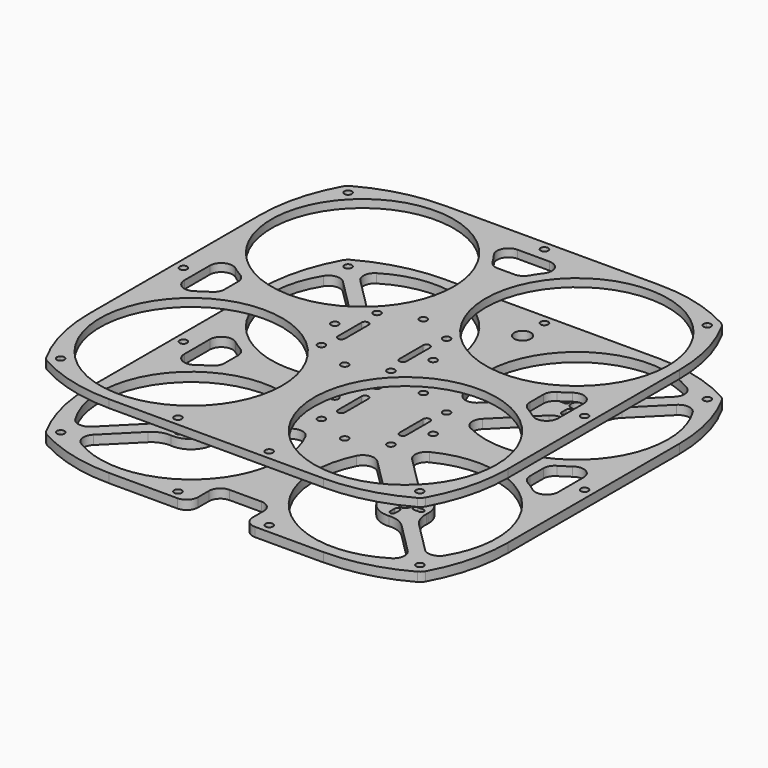
from build123d import *

# Parameters (mm, degrees)
F0_R     = 1.65
F0_W     = 3
F0_H     = 16
F1_DEPTH = 3.5
F2_R     = 5
F3_R     = 5
F4_R     = 1.49999
F6_R     = 1.65
F6_R_2   = 3.65
F6_R_3   = 2.5
F7_DEPTH = 4
F8_R     = 10
F9_R     = 5
F10_R    = 5
F11_R    = 5
F12_R    = 5
F13_R    = 5


# Not quite as in the source:
# - a fillet or chamfer is up to 0.001 mm smaller than in the source, because OpenCascade refuses the exact size


with BuildPart() as f1:
    # F0 (on Top) → F1 (new body)
    with BuildSketch(Plane.XY):
        with BuildLine():
            ThreePointArc((-118.3161303103, 11.4814622591), (-125.7425371815, 24.7657335065), (-128.3161303103, 39.7657335065))
            Line((-128.3161303103, 39.7657335065), (-128.3161303103, -54.2342664935))
            ThreePointArc((-128.3161303103, -54.2342664935), (-125.7425371815, -39.2342664935), (-118.3161303103, -25.949995246))
            Line((-118.3161303103, -25.949995246), (-118.3161303103, 11.4814622591))
        make_face()
        with Locations((-124.3161303103, -7.2342664935)):
            Circle(F0_R, mode=Mode.SUBTRACT)
        with BuildLine():
            ThreePointArc((-110.1359363333, 71.5855377903), (-110.5165386302, 69.6721207263), (-111.6004022776, 68.0500040342))
            ThreePointArc((-111.6004022776, 68.0500040342), (-114.9969936141, 66.587468671), (-118.4695912998, 67.8590455302))
            ThreePointArc((-118.4695912998, 67.8590455302), (-125.7832101753, 54.6501927757), (-128.3161303103, 39.7657335065))
            ThreePointArc((-128.3161303103, 39.7657335065), (-125.7425371815, 24.7657335065), (-118.3161303103, 11.4814622591))
            ThreePointArc((-118.3161303103, 11.4814622591), (-111.4659489145, 4.6575049476), (-103.3161303103, -0.545555235))
            ThreePointArc((-103.3161303103, -0.545555235), (-76.8540279471, -4.7678631711), (-52.6834054177, 6.8015686354))
            ThreePointArc((-52.6834054177, 6.8015686354), (-52.7328564993, 9.1824596955), (-50.3519654391, 9.1330086139))
            ThreePointArc((-50.3519654391, 9.1330086139), (-41.4330345603, 23.3095404353), (-38.3161303103, 39.7657335065))
            ThreePointArc((-38.3161303103, 39.7657335065), (-39.5039859131, 50.0368582413), (-43.0048415688, 59.7657335065))
            ThreePointArc((-43.0048415688, 59.7657335065), (-48.2079017513, 67.9155521107), (-55.0318590628, 74.7657335065))
            ThreePointArc((-55.0318590628, 74.7657335065), (-68.3161303103, 82.1921403777), (-83.3161303103, 84.7657335065))
            ThreePointArc((-83.3161303103, 84.7657335065), (-98.2005907401, 82.2328129648), (-111.4094442555, 74.9191929604))
            ThreePointArc((-111.4094442555, 74.9191929604), (-110.4651515819, 73.3698499281), (-110.1359363333, 71.5855377903))
        make_face()
        with BuildLine():
            ThreePointArc((-111.6004022776, 68.0500040342), (-68.0087934859, 76.7209150018), (-43.3161303103, 39.7657335065))
            ThreePointArc((-43.3161303103, 39.7657335065), (-98.6234671346, 2.8105520113), (-111.6004022776, 68.0500040342))
        make_face(mode=Mode.SUBTRACT)
        with BuildLine():
            ThreePointArc((-52.6834054177, 6.8015686354), (-76.8540279471, -4.7678631711), (-103.3161303103, -0.545555235))
            Line((-103.3161303103, -0.545555235), (-103.3161303103, -13.922977752))
            ThreePointArc((-103.3161303103, -13.922977752), (-76.8540279471, -9.7006698158), (-52.6834054177, -21.2701016223))
            ThreePointArc((-52.6834054177, -21.2701016223), (-50.9031838295, -20.9733058839), (-49.9161303103, -22.4842664935))
            ThreePointArc((-49.9161303103, -22.4842664935), (-50.028945865, -23.0839030345), (-50.3519654391, -23.6015416009))
            ThreePointArc((-50.3519654391, -23.6015416009), (-41.4330345603, -37.7780734222), (-38.3161303103, -54.2342664935))
            ThreePointArc((-38.3161303103, -54.2342664935), (-51.4963251569, -86.0540716469), (-83.3161303103, -99.2342664935))
            Line((-83.3161303103, -99.2342664935), (10.6838696897, -99.2342664935))
            ThreePointArc((10.6838696897, -99.2342664935), (-30.5682370454, -72.2138018022), (-22.2802951815, -23.6015416009))
            ThreePointArc((-22.2802951815, -23.6015416009), (-22.2328564993, -21.3175403045), (-19.9488552029, -21.2701016223))
            ThreePointArc((-19.9488552029, -21.2701016223), (4.2217673265, -9.7006698158), (30.6838696897, -13.922977752))
            Line((30.6838696897, -13.922977752), (30.6838696897, -0.545555235))
            ThreePointArc((30.6838696897, -0.545555235), (4.2217673265, -4.7678631711), (-19.9488552029, 6.8015686354))
            ThreePointArc((-19.9488552029, 6.8015686354), (-22.2328564993, 6.8490073176), (-22.2802951815, 9.1330086139))
            ThreePointArc((-22.2802951815, 9.1330086139), (-33.849726988, 33.3036311434), (-29.6274190518, 59.7657335065))
            Line((-29.6274190518, 59.7657335065), (-43.0048415688, 59.7657335065))
            ThreePointArc((-43.0048415688, 59.7657335065), (-39.5039859131, 50.0368582413), (-38.3161303103, 39.7657335065))
            ThreePointArc((-38.3161303103, 39.7657335065), (-41.4330345603, 23.3095404353), (-50.3519654391, 9.1330086139))
            ThreePointArc((-50.3519654391, 9.1330086139), (-50.028945865, 8.6153700475), (-49.9161303103, 8.0157335065))
            ThreePointArc((-49.9161303103, 8.0157335065), (-50.9031838295, 6.504772897), (-52.6834054177, 6.8015686354))
        make_face()
        with Locations((-56.3161303103, -95.2342664935)):
            Circle(F0_R, mode=Mode.SUBTRACT)
        with Locations((-16.3161303103, -95.2342664935)):
            Circle(F0_R, mode=Mode.SUBTRACT)
        with Locations((-36.3161303103, -28.8010226058)):
            Circle(F0_R, mode=Mode.SUBTRACT)
        with Locations((-57.8828868985, -7.2342664935)):
            Circle(F0_R, mode=Mode.SUBTRACT)
        with Locations((-49.8161303103, -7.2342664935)):
            Rectangle(F0_W, F0_H, mode=Mode.SUBTRACT)
        with Locations((-22.8161303103, -7.2342664935)):
            Rectangle(F0_W, F0_H, mode=Mode.SUBTRACT)
        with Locations((-14.7493727702, -7.2342664935)):
            Circle(F0_R, mode=Mode.SUBTRACT)
        with Locations((-36.3161303103, 14.3324905707)):
            Circle(F0_R, mode=Mode.SUBTRACT)
        with BuildLine():
            ThreePointArc((38.7771836349, 74.9191929604), (25.5683301195, 82.2328129648), (10.6838696897, 84.7657335065))
            ThreePointArc((10.6838696897, 84.7657335065), (-4.3161303103, 82.1921403777), (-17.6004015578, 74.7657335065))
            ThreePointArc((-17.6004015578, 74.7657335065), (-24.4243588693, 67.9155521107), (-29.6274190518, 59.7657335065))
            ThreePointArc((-29.6274190518, 59.7657335065), (-33.849726988, 33.3036311434), (-22.2802951815, 9.1330086139))
            ThreePointArc((-22.2802951815, 9.1330086139), (-20.4664937693, 9.5529179518), (-19.4161303103, 8.0157335065))
            ThreePointArc((-19.4161303103, 8.0157335065), (-19.5551697008, 7.3527870257), (-19.9488552029, 6.8015686354))
            ThreePointArc((-19.9488552029, 6.8015686354), (4.2217673265, -4.7678631711), (30.6838696897, -0.545555235))
            ThreePointArc((30.6838696897, -0.545555235), (38.8336882939, 4.6575049476), (45.6838696897, 11.4814622591))
            ThreePointArc((45.6838696897, 11.4814622591), (53.1102765609, 24.7657335065), (55.6838696897, 39.7657335065))
            ThreePointArc((55.6838696897, 39.7657335065), (53.1509495547, 54.6501927757), (45.8373306792, 67.8590455302))
            ThreePointArc((45.8373306792, 67.8590455302), (42.3647330544, 66.5874686693), (38.9681417432, 68.050003948))
            ThreePointArc((38.9681417432, 68.050003948), (37.5056065855, 71.4465953585), (38.7771836349, 74.9191929604))
        make_face()
        with BuildLine():
            ThreePointArc((50.6838696897, 39.7657335065), (-26.2713118289, 24.4583967385), (38.9681417432, 68.050003948))
            ThreePointArc((38.9681417432, 68.050003948), (47.6390512083, 55.0730702746), (50.6838696897, 39.7657335065))
        make_face(mode=Mode.SUBTRACT)
        with BuildLine():
            Line((55.6838696897, -54.2342664935), (55.6838696897, 39.7657335065))
            ThreePointArc((55.6838696897, 39.7657335065), (53.1102765609, 24.7657335065), (45.6838696897, 11.4814622591))
            Line((45.6838696897, 11.4814622591), (45.6838696897, -25.949995246))
            ThreePointArc((45.6838696897, -25.949995246), (53.1102765609, -39.2342664935), (55.6838696897, -54.2342664935))
        make_face()
        with Locations((51.6838696897, -7.2342664935)):
            Circle(F0_R, mode=Mode.SUBTRACT)
        with BuildLine():
            ThreePointArc((-118.3161303103, -25.949995246), (-125.7425371815, -39.2342664935), (-128.3161303103, -54.2342664935))
            ThreePointArc((-128.3161303103, -54.2342664935), (-125.7832101753, -69.1187257626), (-118.4695912998, -82.3275785171))
            ThreePointArc((-118.4695912998, -82.3275785171), (-114.9969936141, -81.056001658), (-111.6004022776, -82.5185370211))
            ThreePointArc((-111.6004022776, -82.5185370211), (-110.5165386302, -84.1406537133), (-110.1359363333, -86.0540707772))
            ThreePointArc((-110.1359363333, -86.0540707772), (-110.4651515819, -87.8383829151), (-111.4094442555, -89.3877259474))
            ThreePointArc((-111.4094442555, -89.3877259474), (-98.2005907401, -96.7013459517), (-83.3161303103, -99.2342664935))
            ThreePointArc((-83.3161303103, -99.2342664935), (-51.4963251569, -86.0540716469), (-38.3161303103, -54.2342664935))
            ThreePointArc((-38.3161303103, -54.2342664935), (-41.4330345603, -37.7780734222), (-50.3519654391, -23.6015416009))
            ThreePointArc((-50.3519654391, -23.6015416009), (-52.7328564993, -23.6509926824), (-52.6834054177, -21.2701016223))
            ThreePointArc((-52.6834054177, -21.2701016223), (-76.8540279471, -9.7006698158), (-103.3161303103, -13.922977752))
            ThreePointArc((-103.3161303103, -13.922977752), (-111.4659489145, -19.1260379345), (-118.3161303103, -25.949995246))
        make_face()
        with BuildLine():
            ThreePointArc((-43.3161303103, -54.2342664935), (-68.0087934859, -91.1894479887), (-111.6004022776, -82.5185370211))
            ThreePointArc((-111.6004022776, -82.5185370211), (-98.6234671346, -17.2790849982), (-43.3161303103, -54.2342664935))
        make_face(mode=Mode.SUBTRACT)
        with BuildLine():
            ThreePointArc((-22.2802951815, -23.6015416009), (-30.5682370454, -72.2138018022), (10.6838696897, -99.2342664935))
            ThreePointArc((10.6838696897, -99.2342664935), (25.5683301195, -96.7013459517), (38.7771836349, -89.3877259474))
            ThreePointArc((38.7771836349, -89.3877259474), (37.5056065853, -85.9151283522), (38.9681417336, -82.5185369445))
            ThreePointArc((38.9681417336, -82.5185369445), (42.3647330476, -81.0560016565), (45.8373306792, -82.3275785171))
            ThreePointArc((45.8373306792, -82.3275785171), (53.1509495547, -69.1187257626), (55.6838696897, -54.2342664935))
            ThreePointArc((55.6838696897, -54.2342664935), (53.1102765609, -39.2342664935), (45.6838696897, -25.949995246))
            ThreePointArc((45.6838696897, -25.949995246), (38.8336882939, -19.1260379345), (30.6838696897, -13.922977752))
            ThreePointArc((30.6838696897, -13.922977752), (4.2217673265, -9.7006698158), (-19.9488552029, -21.2701016223))
            ThreePointArc((-19.9488552029, -21.2701016223), (-19.5551697008, -21.8213200127), (-19.4161303103, -22.4842664935))
            ThreePointArc((-19.4161303103, -22.4842664935), (-20.4664937693, -24.0214509387), (-22.2802951815, -23.6015416009))
        make_face()
        with BuildLine():
            ThreePointArc((50.6838696897, -54.2342664935), (47.6390512057, -69.5416032678), (38.9681417336, -82.5185369445))
            ThreePointArc((38.9681417336, -82.5185369445), (-26.2713118263, -38.9269297191), (50.6838696897, -54.2342664935))
        make_face(mode=Mode.SUBTRACT)
        with BuildLine():
            Line((10.6838696897, 84.7657335065), (-83.3161303103, 84.7657335065))
            ThreePointArc((-83.3161303103, 84.7657335065), (-68.3161303103, 82.1921403777), (-55.0318590628, 74.7657335065))
            Line((-55.0318590628, 74.7657335065), (-17.6004015578, 74.7657335065))
            ThreePointArc((-17.6004015578, 74.7657335065), (-4.3161303103, 82.1921403777), (10.6838696897, 84.7657335065))
        make_face()
        with Locations((-36.3161303103, 80.7657335065)):
            Circle(F0_R, mode=Mode.SUBTRACT)
        with BuildLine():
            ThreePointArc((-118.4695912998, 67.8590455302), (-114.9969936141, 66.587468671), (-111.6004022776, 68.0500040342))
            ThreePointArc((-111.6004022776, 68.0500040342), (-110.5165386302, 69.6721207263), (-110.1359363333, 71.5855377903))
            ThreePointArc((-110.1359363333, 71.5855377903), (-110.4651515819, 73.3698499281), (-111.4094442555, 74.9191929604))
            ThreePointArc((-111.4094442555, 74.9191929604), (-112.6991130718, 73.8485785175), (-113.9480162869, 72.7306779403))
            ThreePointArc((-113.9480162869, 72.7306779403), (-113.6058108358, 72.202964678), (-113.4859363333, 71.5855377903))
            ThreePointArc((-113.4859363333, 71.5855377903), (-114.4905609156, 70.0669889533), (-116.2810764184, 70.3976176812))
            ThreePointArc((-116.2810764184, 70.3976176812), (-117.3989769273, 69.148714405), (-118.4695912998, 67.8590455302))
        make_face()
        with BuildLine():
            ThreePointArc((-117.5473543924, 75.9656134682), (-114.2956364532, 76.5144216509), (-111.4094442555, 74.9191929604))
            ThreePointArc((-111.4094442555, 74.9191929604), (-98.2005907401, 82.2328129648), (-83.3161303103, 84.7657335065))
            ThreePointArc((-83.3161303103, 84.7657335065), (-100.9882751635, 82.5305075258), (-117.5473543924, 75.9656134682))
        make_face()
        with BuildLine():
            ThreePointArc((-119.516012195, 73.9969555156), (-120.064820139, 70.7452375877), (-118.4695912998, 67.8590455302))
            ThreePointArc((-118.4695912998, 67.8590455302), (-117.3989769273, 69.148714405), (-116.2810764184, 70.3976176812))
            ThreePointArc((-116.2810764184, 70.3976176812), (-116.3026625542, 72.7522639473), (-113.9480162869, 72.7306779403))
            ThreePointArc((-113.9480162869, 72.7306779403), (-112.6991130718, 73.8485785175), (-111.4094442555, 74.9191929604))
            ThreePointArc((-111.4094442555, 74.9191929604), (-114.2956364532, 76.5144216509), (-117.5473543924, 75.9656134682))
            ThreePointArc((-117.5473543924, 75.9656134682), (-118.671470374, 75.1210715615), (-119.516012195, 73.9969555156))
        make_face()
        with BuildLine():
            ThreePointArc((-128.3161303103, 39.7657335065), (-125.7832101753, 54.6501927757), (-118.4695912998, 67.8590455302))
            ThreePointArc((-118.4695912998, 67.8590455302), (-120.064820139, 70.7452375877), (-119.516012195, 73.9969555156))
            ThreePointArc((-119.516012195, 73.9969555156), (-126.0809048288, 57.4378771164), (-128.3161303103, 39.7657335065))
        make_face()
        with BuildLine():
            ThreePointArc((55.6838696897, 39.7657335065), (53.4486442082, 57.4378771164), (46.8837515744, 73.9969555156))
            ThreePointArc((46.8837515744, 73.9969555156), (47.3462153, 72.8304515808), (47.5036757128, 71.5855377903))
            ThreePointArc((47.5036757128, 71.5855377903), (47.0681184406, 69.5444933067), (45.8373306792, 67.8590455302))
            ThreePointArc((45.8373306792, 67.8590455302), (53.1509495547, 54.6501927757), (55.6838696897, 39.7657335065))
        make_face()
        with BuildLine():
            ThreePointArc((44.9150937718, 75.9656134682), (41.6633758326, 76.5144216509), (38.7771836349, 74.9191929604))
            ThreePointArc((38.7771836349, 74.9191929604), (40.0668524512, 73.8485785175), (41.3157556663, 72.7306779403))
            ThreePointArc((41.3157556663, 72.7306779403), (43.1211026004, 73.1156632879), (44.1536757128, 71.5855377903))
            ThreePointArc((44.1536757128, 71.5855377903), (44.0222245497, 70.9401623725), (43.6488157978, 70.3976176812))
            ThreePointArc((43.6488157978, 70.3976176812), (44.7667163068, 69.148714405), (45.8373306792, 67.8590455302))
            ThreePointArc((45.8373306792, 67.8590455302), (47.0681184406, 69.5444933067), (47.5036757128, 71.5855377903))
            ThreePointArc((47.5036757128, 71.5855377903), (47.3462153, 72.8304515808), (46.8837515744, 73.9969555156))
            ThreePointArc((46.8837515744, 73.9969555156), (46.0392097534, 75.1210715615), (44.9150937718, 75.9656134682))
        make_face()
        with BuildLine():
            ThreePointArc((44.9150937718, 75.9656134682), (28.3560145429, 82.5305075258), (10.6838696897, 84.7657335065))
            ThreePointArc((10.6838696897, 84.7657335065), (25.5683301195, 82.2328129648), (38.7771836349, 74.9191929604))
            ThreePointArc((38.7771836349, 74.9191929604), (41.6633758326, 76.5144216509), (44.9150937718, 75.9656134682))
        make_face()
        with BuildLine():
            ThreePointArc((41.3157556663, 72.7306779403), (40.0668524512, 73.8485785175), (38.7771836349, 74.9191929604))
            ThreePointArc((38.7771836349, 74.9191929604), (37.5056065855, 71.4465953585), (38.9681417432, 68.050003948))
            ThreePointArc((38.9681417432, 68.050003948), (42.3647330544, 66.5874686693), (45.8373306792, 67.8590455302))
            ThreePointArc((45.8373306792, 67.8590455302), (44.7667163068, 69.148714405), (43.6488157978, 70.3976176812))
            ThreePointArc((43.6488157978, 70.3976176812), (41.3369494919, 70.4188116332), (41.3157556663, 72.7306779403))
        make_face()
        with BuildLine():
            ThreePointArc((41.3157556663, -87.1992109272), (40.0668524512, -88.3171115044), (38.7771836349, -89.3877259474))
            ThreePointArc((38.7771836349, -89.3877259474), (41.6633758326, -90.9829546378), (44.9150937718, -90.4341464552))
            ThreePointArc((44.9150937718, -90.4341464552), (46.0392097534, -89.5896045485), (46.8837515744, -88.4654885026))
            ThreePointArc((46.8837515744, -88.4654885026), (47.3462153, -87.2989845677), (47.5036757128, -86.0540707772))
            ThreePointArc((47.5036757128, -86.0540707772), (47.0681184406, -84.0130262937), (45.8373306792, -82.3275785171))
            ThreePointArc((45.8373306792, -82.3275785171), (44.7667163068, -83.6172473919), (43.6488157978, -84.8661506681))
            ThreePointArc((43.6488157978, -84.8661506681), (44.0222245497, -85.4086953595), (44.1536757128, -86.0540707772))
            ThreePointArc((44.1536757128, -86.0540707772), (43.1211026004, -87.5841962748), (41.3157556663, -87.1992109272))
        make_face()
        with BuildLine():
            ThreePointArc((46.8837515744, -88.4654885026), (53.4486442082, -71.9064101034), (55.6838696897, -54.2342664935))
            ThreePointArc((55.6838696897, -54.2342664935), (53.1509495547, -69.1187257626), (45.8373306792, -82.3275785171))
            ThreePointArc((45.8373306792, -82.3275785171), (47.0681184406, -84.0130262937), (47.5036757128, -86.0540707772))
            ThreePointArc((47.5036757128, -86.0540707772), (47.3462153, -87.2989845677), (46.8837515744, -88.4654885026))
        make_face()
        with BuildLine():
            ThreePointArc((38.9681417336, -82.5185369445), (37.5056065853, -85.9151283522), (38.7771836349, -89.3877259474))
            ThreePointArc((38.7771836349, -89.3877259474), (40.0668524512, -88.3171115044), (41.3157556663, -87.1992109272))
            ThreePointArc((41.3157556663, -87.1992109272), (41.3369494919, -84.8873446201), (43.6488157978, -84.8661506681))
            ThreePointArc((43.6488157978, -84.8661506681), (44.7667163068, -83.6172473919), (45.8373306792, -82.3275785171))
            ThreePointArc((45.8373306792, -82.3275785171), (42.3647330476, -81.0560016565), (38.9681417336, -82.5185369445))
        make_face()
        with BuildLine():
            ThreePointArc((38.7771836349, -89.3877259474), (25.5683301195, -96.7013459517), (10.6838696897, -99.2342664935))
            ThreePointArc((10.6838696897, -99.2342664935), (28.3560145429, -96.9990405127), (44.9150937718, -90.4341464552))
            ThreePointArc((44.9150937718, -90.4341464552), (41.6633758326, -90.9829546378), (38.7771836349, -89.3877259474))
        make_face()
        with BuildLine():
            ThreePointArc((-111.4094442555, -89.3877259474), (-114.2956364532, -90.9829546378), (-117.5473543924, -90.4341464552))
            ThreePointArc((-117.5473543924, -90.4341464552), (-100.9882751635, -96.9990405127), (-83.3161303103, -99.2342664935))
            ThreePointArc((-83.3161303103, -99.2342664935), (-98.2005907401, -96.7013459517), (-111.4094442555, -89.3877259474))
        make_face()
        with BuildLine():
            ThreePointArc((-116.2810764184, -84.8661506681), (-117.3989769273, -83.6172473919), (-118.4695912998, -82.3275785171))
            ThreePointArc((-118.4695912998, -82.3275785171), (-120.064820139, -85.2137705746), (-119.516012195, -88.4654885026))
            ThreePointArc((-119.516012195, -88.4654885026), (-118.671470374, -89.5896045485), (-117.5473543924, -90.4341464552))
            ThreePointArc((-117.5473543924, -90.4341464552), (-114.2956364532, -90.9829546378), (-111.4094442555, -89.3877259474))
            ThreePointArc((-111.4094442555, -89.3877259474), (-112.6991130718, -88.3171115044), (-113.9480162869, -87.1992109272))
            ThreePointArc((-113.9480162869, -87.1992109272), (-116.3026625542, -87.2207969343), (-116.2810764184, -84.8661506681))
        make_face()
        with BuildLine():
            ThreePointArc((-111.6004022776, -82.5185370211), (-114.9969936141, -81.056001658), (-118.4695912998, -82.3275785171))
            ThreePointArc((-118.4695912998, -82.3275785171), (-117.3989769273, -83.6172473919), (-116.2810764184, -84.8661506681))
            ThreePointArc((-116.2810764184, -84.8661506681), (-114.4905609156, -84.5355219403), (-113.4859363333, -86.0540707772))
            ThreePointArc((-113.4859363333, -86.0540707772), (-113.6058108358, -86.6714976649), (-113.9480162869, -87.1992109272))
            ThreePointArc((-113.9480162869, -87.1992109272), (-112.6991130718, -88.3171115044), (-111.4094442555, -89.3877259474))
            ThreePointArc((-111.4094442555, -89.3877259474), (-110.4651515819, -87.8383829151), (-110.1359363333, -86.0540707772))
            ThreePointArc((-110.1359363333, -86.0540707772), (-110.5165386302, -84.1406537133), (-111.6004022776, -82.5185370211))
        make_face()
        with BuildLine():
            ThreePointArc((-118.4695912998, -82.3275785171), (-125.7832101753, -69.1187257626), (-128.3161303103, -54.2342664935))
            ThreePointArc((-128.3161303103, -54.2342664935), (-126.0809048288, -71.9064101034), (-119.516012195, -88.4654885026))
            ThreePointArc((-119.516012195, -88.4654885026), (-120.064820139, -85.2137705746), (-118.4695912998, -82.3275785171))
        make_face()
    extrude(amount=F1_DEPTH)

    # F2
    f2_edges = [f1.edges().sort_by_distance(p)[0] for p in [
        (-118.31613, 11.481462, 1.75),
        (45.68387, 11.481462, 1.75),
        (45.68387, -25.949995, 1.75),
        (-118.31613, -25.949995, 1.75),
        (-17.600402, 74.765734, 1.75),
        (-55.031859, 74.765734, 1.75),
    ]]
    fillet(f2_edges, radius=F2_R)

    # F3
    f3_edges = [f1.edges().sort_by_distance(p)[0] for p in [
        (30.68387, -0.545555, 1.75),
        (30.68387, -13.922978, 1.75),
        (-103.31613, -0.545555, 1.75),
        (-103.31613, -13.922978, 1.75),
        (-29.627419, 59.765734, 1.75),
        (-43.004842, 59.765734, 1.75),
    ]]
    fillet(f3_edges, radius=F3_R)

    # F4 (radius 1.5 in the source; OpenCascade refuses exactly that, so slightly less here)
    f4_edges = [f1.edges().sort_by_distance(p)[0] for p in [
        (-51.31613, -15.234266, 1.75),
        (-24.31613, -15.234266, 1.75),
        (-48.31613, -15.234266, 1.75),
        (-21.31613, -15.234266, 1.75),
        (-24.31613, 0.765734, 1.75),
        (-51.31613, 0.765734, 1.75),
        (-21.31613, 0.765734, 1.75),
        (-48.31613, 0.765734, 1.75),
    ]]
    fillet(f4_edges, radius=F4_R)


with BuildPart() as f7:
    # F6 (on offset) → F7 (new body)
    with BuildSketch(Plane(origin=(0, 0, -25), x_dir=(1, 0, 0), z_dir=(0, 0, -1))):
        with BuildLine():
            ThreePointArc((-110.3161303103, 18.2342664935), (-123.5653539053, 34.109654696), (-128.3161303103, 54.2342664935))
            Line((-128.3161303103, 54.2342664935), (-128.3161303103, -39.7657335065))
            ThreePointArc((-128.3161303103, -39.7657335065), (-126.0809048288, -57.4378771164), (-119.516012195, -73.9969555156))
            ThreePointArc((-119.516012195, -73.9969555156), (-118.1392463202, -67.5880224216), (-111.6004023308, -68.0500039809))
            ThreePointArc((-111.6004023308, -68.0500039809), (-110.5165386447, -69.6721206915), (-110.1359363333, -71.5855377903))
            ThreePointArc((-110.1359363333, -71.5855377903), (-112.5920309003, -75.8900174508), (-117.5473543924, -75.9656134682))
            ThreePointArc((-117.5473543924, -75.9656134682), (-100.9882751635, -82.5305075258), (-83.3161303103, -84.7657335065))
            Line((-83.3161303103, -84.7657335065), (10.6838696897, -84.7657335065))
            ThreePointArc((10.6838696897, -84.7657335065), (28.3560145429, -82.5305075258), (44.9150937718, -75.9656134682))
            ThreePointArc((44.9150937718, -75.9656134682), (38.5061605306, -74.5888480254), (38.9681417336, -68.0500039576))
            ThreePointArc((38.9681417336, -68.0500039576), (44.4170928267, -66.9661401079), (47.5036757128, -71.5855377903))
            ThreePointArc((47.5036757128, -71.5855377903), (47.3462153, -72.8304515808), (46.8837515744, -73.9969555156))
            ThreePointArc((46.8837515744, -73.9969555156), (53.4486442082, -57.4378771164), (55.6838696897, -39.7657335065))
            Line((55.6838696897, -39.7657335065), (55.6838696897, 54.2342664935))
            ThreePointArc((55.6838696897, 54.2342664935), (53.1509495547, 69.1187257626), (45.8373306792, 82.3275785171))
            ThreePointArc((45.8373306792, 82.3275785171), (42.364732999, 81.0560016578), (38.9681416648, 82.5185370133))
            ThreePointArc((38.9681416648, 82.5185370133), (37.505606584, 85.9151284009), (38.7771836349, 89.3877259474))
            ThreePointArc((38.7771836349, 89.3877259474), (25.5683301195, 96.7013459517), (10.6838696897, 99.2342664935))
            Line((10.6838696897, 99.2342664935), (-24.3161303103, 99.2342664935))
            Line((-24.3161303103, 99.2342664935), (-24.3161303103, 83.2342664935))
            Line((-24.3161303103, 83.2342664935), (-36.3161303103, 83.2342664935))
            Line((-36.3161303103, 83.2342664935), (-48.3161303103, 83.2342664935))
            Line((-48.3161303103, 83.2342664935), (-48.3161303103, 99.2342664935))
            Line((-48.3161303103, 99.2342664935), (-83.3161303103, 99.2342664935))
            ThreePointArc((-83.3161303103, 99.2342664935), (-51.4963251569, 86.0540716469), (-38.3161303103, 54.2342664935))
            ThreePointArc((-38.3161303103, 54.2342664935), (-41.4330345603, 37.7780734222), (-50.3519654391, 23.6015416009))
            ThreePointArc((-50.3519654391, 23.6015416009), (-50.028945865, 23.0839030345), (-49.9161303103, 22.4842664935))
            ThreePointArc((-49.9161303103, 22.4842664935), (-50.9031838295, 20.9733058839), (-52.6834054177, 21.2701016223))
            ThreePointArc((-52.6834054177, 21.2701016223), (-78.2608112683, 9.5191264469), (-105.8161303103, 15.2631233232))
            ThreePointArc((-105.8161303103, 15.2631233232), (-103.9860032914, 13.4329963042), (-103.3161303103, 10.9329963042))
            Line((-103.3161303103, 10.9329963042), (-103.3161303103, 3.5355366827))
            ThreePointArc((-103.3161303103, 3.5355366827), (-103.9860032914, 1.0355366827), (-105.8161303103, -0.7945903362))
            ThreePointArc((-105.8161303103, -0.7945903362), (-108.1106745274, -2.2126966511), (-110.3161303103, -3.7657335065))
            ThreePointArc((-110.3161303103, -3.7657335065), (-115.5521982878, -4.2378694615), (-118.3161303103, 0.2342664935))
            Line((-118.3161303103, 0.2342664935), (-118.3161303103, 14.2342664935))
            ThreePointArc((-118.3161303103, 14.2342664935), (-115.5521982878, 18.7064024485), (-110.3161303103, 18.2342664935))
        make_face()
        with BuildLine():
            ThreePointArc((-109.3994195191, -70.0916634024), (-110.5190717285, -69.091489732), (-111.6004023308, -68.0500039809))
            ThreePointArc((-111.6004023308, -68.0500039809), (-112.6418872793, -66.9686741232), (-113.6420602062, -65.8490227153))
            ThreePointArc((-113.6420602062, -65.8490227153), (-112.647698019, -12.5690584202), (-59.5945080892, -7.5588299112))
            ThreePointArc((-59.5945080892, -7.5588299112), (-55.0318590628, -11.4814622591), (-51.109226715, -16.0441112854))
            ThreePointArc((-51.109226715, -16.0441112854), (-45.3143136181, -27.2812660332), (-43.3161303103, -39.7657335065))
            ThreePointArc((-43.3161303103, -39.7657335065), (-66.6327788537, -76.120455128), (-109.3994195191, -70.0916634024))
        make_face(mode=Mode.SUBTRACT)
        with Locations((-51.5661303103, -8.0157335065)):
            Circle(F6_R, mode=Mode.SUBTRACT)
        with Locations((-57.8828868985, 7.2342664935)):
            Circle(F6_R, mode=Mode.SUBTRACT)
        with Locations((-36.3161303103, -80.7657335065)):
            Circle(F6_R, mode=Mode.SUBTRACT)
        with Locations((-36.3161303103, -68.7657335065)):
            Circle(F6_R_2, mode=Mode.SUBTRACT)
        with BuildLine():
            ThreePointArc((41.0097995856, -65.8490227153), (40.0096266699, -66.9686741111), (38.9681417336, -68.0500039576))
            ThreePointArc((38.9681417336, -68.0500039576), (37.88681112, -69.0914897208), (36.7671588985, -70.0916634024))
            ThreePointArc((36.7671588985, -70.0916634024), (-16.5128053966, -69.0973012153), (-21.5230339056, -16.0441112854))
            ThreePointArc((-21.5230339056, -16.0441112854), (-17.6004015578, -11.4814622591), (-13.0377525314, -7.5588299112))
            ThreePointArc((-13.0377525314, -7.5588299112), (28.7273603602, -4.0665396162), (50.6838696897, -39.7657335065))
            ThreePointArc((50.6838696897, -39.7657335065), (48.1874508243, -53.6754927454), (41.0097995856, -65.8490227153))
        make_face(mode=Mode.SUBTRACT)
        with Locations((-36.3161303103, -14.3324905707)):
            Circle(F6_R, mode=Mode.SUBTRACT)
        with Locations((-21.0661303103, -8.0157335065)):
            Circle(F6_R, mode=Mode.SUBTRACT)
        with Locations((-14.7493727702, 7.2342664935)):
            Circle(F6_R, mode=Mode.SUBTRACT)
        with Locations((51.6838696897, 7.2342664935)):
            Circle(F6_R, mode=Mode.SUBTRACT)
        with Locations((-124.3161303103, 7.2342664935)):
            Circle(F6_R, mode=Mode.SUBTRACT)
        with BuildLine():
            ThreePointArc((-51.3161303103, 13.7342664935), (-49.8161303103, 15.2342664935), (-48.3161303103, 13.7342664935))
            Line((-48.3161303103, 13.7342664935), (-48.3161303103, 0.7342664935))
            ThreePointArc((-48.3161303103, 0.7342664935), (-49.8161303103, -0.7657335065), (-51.3161303103, 0.7342664935))
            Line((-51.3161303103, 0.7342664935), (-51.3161303103, 13.7342664935))
        make_face(mode=Mode.SUBTRACT)
        with Locations((-56.3161303103, 95.2342664935)):
            Circle(F6_R, mode=Mode.SUBTRACT)
        with BuildLine():
            ThreePointArc((-24.3161303103, 13.7342664935), (-22.8161303103, 15.2342664935), (-21.3161303103, 13.7342664935))
            Line((-21.3161303103, 13.7342664935), (-21.3161303103, 0.7342664935))
            ThreePointArc((-21.3161303103, 0.7342664935), (-22.8161303103, -0.7657335065), (-24.3161303103, 0.7342664935))
            Line((-24.3161303103, 0.7342664935), (-24.3161303103, 13.7342664935))
        make_face(mode=Mode.SUBTRACT)
        with Locations((-36.3161303103, 28.8010226058)):
            Circle(F6_R, mode=Mode.SUBTRACT)
        with Locations((-21.0661303103, 22.4842664935)):
            Circle(F6_R, mode=Mode.SUBTRACT)
        with BuildLine():
            ThreePointArc((37.6838696897, 18.2342664935), (42.9199376672, 18.7064024485), (45.6838696897, 14.2342664935))
            Line((45.6838696897, 14.2342664935), (45.6838696897, 0.2342664935))
            ThreePointArc((45.6838696897, 0.2342664935), (42.9199376672, -4.2378694615), (37.6838696897, -3.7657335065))
            ThreePointArc((37.6838696897, -3.7657335065), (35.4784139068, -2.2126966511), (33.1838696897, -0.7945903362))
            ThreePointArc((33.1838696897, -0.7945903362), (31.3537426708, 1.0355366827), (30.6838696897, 3.5355366827))
            Line((30.6838696897, 3.5355366827), (30.6838696897, 10.9329963042))
            ThreePointArc((30.6838696897, 10.9329963042), (31.3537426708, 13.4329963042), (33.1838696897, 15.2631233232))
            ThreePointArc((33.1838696897, 15.2631233232), (35.4784139068, 16.681229638), (37.6838696897, 18.2342664935))
        make_face(mode=Mode.SUBTRACT)
        with Locations((-16.3161303103, 95.2342664935)):
            Circle(F6_R, mode=Mode.SUBTRACT)
        with BuildLine():
            ThreePointArc((36.7671588985, 84.5601963894), (37.8868110844, 83.5600227408), (38.9681416648, 82.5185370133))
            ThreePointArc((38.9681416648, 82.5185370133), (40.0096266368, 81.4372071337), (41.0097995856, 80.3175557023))
            ThreePointArc((41.0097995856, 80.3175557023), (48.1874508243, 68.1440257323), (50.6838696897, 54.2342664935))
            ThreePointArc((50.6838696897, 54.2342664935), (28.7273603602, 18.5350726031), (-13.0377525314, 22.0273628981))
            ThreePointArc((-13.0377525314, 22.0273628981), (-17.6004015578, 25.949995246), (-21.5230339056, 30.5126442724))
            ThreePointArc((-21.5230339056, 30.5126442724), (-16.5128053966, 83.5658342022), (36.7671588985, 84.5601963894))
        make_face(mode=Mode.SUBTRACT)
        with BuildLine():
            ThreePointArc((-118.4695912998, 82.3275785171), (-125.7832101753, 69.1187257626), (-128.3161303103, 54.2342664935))
            ThreePointArc((-128.3161303103, 54.2342664935), (-123.5653539053, 34.109654696), (-110.3161303103, 18.2342664935))
            ThreePointArc((-110.3161303103, 18.2342664935), (-108.1106745274, 16.681229638), (-105.8161303103, 15.2631233232))
            ThreePointArc((-105.8161303103, 15.2631233232), (-78.2608112683, 9.5191264469), (-52.6834054177, 21.2701016223))
            ThreePointArc((-52.6834054177, 21.2701016223), (-52.7328564993, 23.6509926824), (-50.3519654391, 23.6015416009))
            ThreePointArc((-50.3519654391, 23.6015416009), (-41.4330345603, 37.7780734222), (-38.3161303103, 54.2342664935))
            ThreePointArc((-38.3161303103, 54.2342664935), (-51.4963251569, 86.0540716469), (-83.3161303103, 99.2342664935))
            ThreePointArc((-83.3161303103, 99.2342664935), (-98.2005907401, 96.7013459517), (-111.4094442555, 89.3877259474))
            ThreePointArc((-111.4094442555, 89.3877259474), (-110.4651515819, 87.8383829151), (-110.1359363333, 86.0540707772))
            ThreePointArc((-110.1359363333, 86.0540707772), (-110.5165386423, 84.1406536843), (-111.6004023219, 82.5185369767))
            ThreePointArc((-111.6004023219, 82.5185369767), (-114.9969936454, 81.0560016571), (-118.4695912998, 82.3275785171))
        make_face()
        with BuildLine():
            ThreePointArc((-113.6420602062, 80.3175557023), (-112.641887275, 81.4372071148), (-111.6004023219, 82.5185369767))
            ThreePointArc((-111.6004023219, 82.5185369767), (-110.5190717239, 83.5600227232), (-109.3994195191, 84.5601963894))
            ThreePointArc((-109.3994195191, 84.5601963894), (-66.6327788537, 90.588988115), (-43.3161303103, 54.2342664935))
            ThreePointArc((-43.3161303103, 54.2342664935), (-45.3143136181, 41.7497990201), (-51.109226715, 30.5126442724))
            ThreePointArc((-51.109226715, 30.5126442724), (-55.0318590628, 25.949995246), (-59.5945080892, 22.0273628981))
            ThreePointArc((-59.5945080892, 22.0273628981), (-112.647698019, 27.0375914072), (-113.6420602062, 80.3175557023))
        make_face(mode=Mode.SUBTRACT)
        with BuildLine():
            Line((0.7843747531, 52.8200529311), (-21.5230339056, 30.5126442724))
            ThreePointArc((-21.5230339056, 30.5126442724), (-17.6004015578, 25.949995246), (-13.0377525314, 22.0273628981))
            Line((-13.0377525314, 22.0273628981), (9.2696561273, 44.3347715569))
            ThreePointArc((9.2696561273, 44.3347715569), (3.6128018778, 47.1631986816), (0.7843747531, 52.8200529311))
        make_face()
        with BuildLine():
            Line((-81.9019167479, 44.3347715569), (-59.5945080892, 22.0273628981))
            ThreePointArc((-59.5945080892, 22.0273628981), (-55.0318590628, 25.949995246), (-51.109226715, 30.5126442724))
            Line((-51.109226715, 30.5126442724), (-73.4166353737, 52.8200529311))
            ThreePointArc((-73.4166353737, 52.8200529311), (-76.2450624984, 47.1631986816), (-81.9019167479, 44.3347715569))
        make_face()
        with BuildLine():
            ThreePointArc((-51.109226715, -16.0441112854), (-55.0318590628, -11.4814622591), (-59.5945080892, -7.5588299112))
            Line((-59.5945080892, -7.5588299112), (-81.9019167479, -29.8662385699))
            ThreePointArc((-81.9019167479, -29.8662385699), (-76.2450624984, -32.6946656947), (-73.4166353737, -38.3515199442))
            Line((-73.4166353737, -38.3515199442), (-51.109226715, -16.0441112854))
        make_face()
        with BuildLine():
            ThreePointArc((-13.0377525314, -7.5588299112), (-17.6004015578, -11.4814622591), (-21.5230339056, -16.0441112854))
            Line((-21.5230339056, -16.0441112854), (0.7843747531, -38.3515199442))
            ThreePointArc((0.7843747531, -38.3515199442), (3.6128018778, -32.6946656947), (9.2696561273, -29.8662385699))
            Line((9.2696561273, -29.8662385699), (-13.0377525314, -7.5588299112))
        make_face()
        with BuildLine():
            ThreePointArc((20.6838696897, 54.2342664935), (20.3964103267, 56.61471905), (19.5505588149, 58.8583149315))
            ThreePointArc((19.5505588149, 58.8583149315), (17.7549375016, 61.3053343053), (15.3079181278, 63.1009556186))
            ThreePointArc((15.3079181278, 63.1009556186), (4.9061691127, 62.3962623304), (0.7843747531, 52.8200529311))
            ThreePointArc((0.7843747531, 52.8200529311), (3.6128018778, 47.1631986816), (9.2696561273, 44.3347715569))
            ThreePointArc((9.2696561273, 44.3347715569), (17.2358871033, 46.6797269435), (20.6838696897, 54.2342664935))
        make_face()
        with BuildLine():
            Line((11.7838696897, 49.7342664935), (11.7838696897, 47.2342664935))
            ThreePointArc((11.7838696897, 47.2342664935), (10.6838696897, 46.1342664935), (9.5838696897, 47.2342664935))
            Line((9.5838696897, 47.2342664935), (9.5838696897, 49.7342664935))
            ThreePointArc((9.5838696897, 49.7342664935), (10.6838696897, 50.8342664935), (11.7838696897, 49.7342664935))
        make_face(mode=Mode.SUBTRACT)
        with BuildLine():
            ThreePointArc((6.1838696897, 55.3342664935), (6.961687149, 55.0120839528), (7.2838696897, 54.2342664935))
            ThreePointArc((7.2838696897, 54.2342664935), (6.961687149, 53.4564490342), (6.1838696897, 53.1342664935))
            Line((6.1838696897, 53.1342664935), (3.6838696897, 53.1342664935))
            ThreePointArc((3.6838696897, 53.1342664935), (2.5838696897, 54.2342664935), (3.6838696897, 55.3342664935))
            Line((3.6838696897, 55.3342664935), (6.1838696897, 55.3342664935))
        make_face(mode=Mode.SUBTRACT)
        with Locations((10.6838696897, 54.2342664935)):
            Circle(F6_R_3, mode=Mode.SUBTRACT)
        with BuildLine():
            Line((15.1838696897, 55.3342664935), (17.6838696897, 55.3342664935))
            ThreePointArc((17.6838696897, 55.3342664935), (18.461687149, 55.0120839528), (18.7838696897, 54.2342664935))
            ThreePointArc((18.7838696897, 54.2342664935), (18.461687149, 53.4564490342), (17.6838696897, 53.1342664935))
            Line((17.6838696897, 53.1342664935), (15.1838696897, 53.1342664935))
            ThreePointArc((15.1838696897, 53.1342664935), (14.0838696897, 54.2342664935), (15.1838696897, 55.3342664935))
        make_face(mode=Mode.SUBTRACT)
        with BuildLine():
            Line((11.7838696897, 61.2342664935), (11.7838696897, 58.7342664935))
            ThreePointArc((11.7838696897, 58.7342664935), (10.6838696897, 57.6342664935), (9.5838696897, 58.7342664935))
            Line((9.5838696897, 58.7342664935), (9.5838696897, 61.2342664935))
            ThreePointArc((9.5838696897, 61.2342664935), (10.6838696897, 62.3342664935), (11.7838696897, 61.2342664935))
        make_face(mode=Mode.SUBTRACT)
        with BuildLine():
            ThreePointArc((-73.3161303103, 54.2342664935), (-78.1315611084, 62.7853039855), (-87.9401787484, 63.1009556186))
            ThreePointArc((-87.9401787484, 63.1009556186), (-90.3871981222, 61.3053343053), (-92.1828194355, 58.8583149315))
            ThreePointArc((-92.1828194355, 58.8583149315), (-91.4781261473, 48.4565659165), (-81.9019167479, 44.3347715569))
            ThreePointArc((-81.9019167479, 44.3347715569), (-76.2450624984, 47.1631986816), (-73.4166353737, 52.8200529311))
            ThreePointArc((-73.4166353737, 52.8200529311), (-73.3412882222, 53.5253762926), (-73.3161303103, 54.2342664935))
        make_face()
        with BuildLine():
            ThreePointArc((-82.2161303103, 47.2342664935), (-83.3161303103, 46.1342664935), (-84.4161303103, 47.2342664935))
            Line((-84.4161303103, 47.2342664935), (-84.4161303103, 49.7342664935))
            ThreePointArc((-84.4161303103, 49.7342664935), (-83.3161303103, 50.8342664935), (-82.2161303103, 49.7342664935))
            Line((-82.2161303103, 49.7342664935), (-82.2161303103, 47.2342664935))
        make_face(mode=Mode.SUBTRACT)
        with BuildLine():
            ThreePointArc((-87.8161303103, 55.3342664935), (-87.038312851, 55.0120839528), (-86.7161303103, 54.2342664935))
            ThreePointArc((-86.7161303103, 54.2342664935), (-87.038312851, 53.4564490342), (-87.8161303103, 53.1342664935))
            Line((-87.8161303103, 53.1342664935), (-90.3161303103, 53.1342664935))
            ThreePointArc((-90.3161303103, 53.1342664935), (-91.4161303103, 54.2342664935), (-90.3161303103, 55.3342664935))
            Line((-90.3161303103, 55.3342664935), (-87.8161303103, 55.3342664935))
        make_face(mode=Mode.SUBTRACT)
        with Locations((-83.3161303103, 54.2342664935)):
            Circle(F6_R_3, mode=Mode.SUBTRACT)
        with BuildLine():
            ThreePointArc((-84.4161303103, 61.2342664935), (-83.3161303103, 62.3342664935), (-82.2161303103, 61.2342664935))
            Line((-82.2161303103, 61.2342664935), (-82.2161303103, 58.7342664935))
            ThreePointArc((-82.2161303103, 58.7342664935), (-83.3161303103, 57.6342664935), (-84.4161303103, 58.7342664935))
            Line((-84.4161303103, 58.7342664935), (-84.4161303103, 61.2342664935))
        make_face(mode=Mode.SUBTRACT)
        with BuildLine():
            ThreePointArc((-75.2161303103, 54.2342664935), (-75.538312851, 53.4564490342), (-76.3161303103, 53.1342664935))
            Line((-76.3161303103, 53.1342664935), (-78.8161303103, 53.1342664935))
            ThreePointArc((-78.8161303103, 53.1342664935), (-79.9161303103, 54.2342664935), (-78.8161303103, 55.3342664935))
            Line((-78.8161303103, 55.3342664935), (-76.3161303103, 55.3342664935))
            ThreePointArc((-76.3161303103, 55.3342664935), (-75.538312851, 55.0120839528), (-75.2161303103, 54.2342664935))
        make_face(mode=Mode.SUBTRACT)
        with BuildLine():
            ThreePointArc((-81.9019167479, -29.8662385699), (-91.4781261473, -33.9880329295), (-92.1828194355, -44.3897819446))
            ThreePointArc((-92.1828194355, -44.3897819446), (-90.3871981222, -46.8368013184), (-87.9401787484, -48.6324226317))
            ThreePointArc((-87.9401787484, -48.6324226317), (-78.1315611084, -48.3167709986), (-73.3161303103, -39.7657335065))
            ThreePointArc((-73.3161303103, -39.7657335065), (-73.3412882222, -39.0568433056), (-73.4166353737, -38.3515199442))
            ThreePointArc((-73.4166353737, -38.3515199442), (-76.2450624984, -32.6946656947), (-81.9019167479, -29.8662385699))
        make_face()
        with BuildLine():
            Line((-82.2161303103, -44.2657335065), (-82.2161303103, -46.7657335065))
            ThreePointArc((-82.2161303103, -46.7657335065), (-83.3161303103, -47.8657335065), (-84.4161303103, -46.7657335065))
            Line((-84.4161303103, -46.7657335065), (-84.4161303103, -44.2657335065))
            ThreePointArc((-84.4161303103, -44.2657335065), (-83.3161303103, -43.1657335065), (-82.2161303103, -44.2657335065))
        make_face(mode=Mode.SUBTRACT)
        with BuildLine():
            Line((-90.3161303103, -38.6657335065), (-87.8161303103, -38.6657335065))
            ThreePointArc((-87.8161303103, -38.6657335065), (-87.038312851, -38.9879160472), (-86.7161303103, -39.7657335065))
            ThreePointArc((-86.7161303103, -39.7657335065), (-87.038312851, -40.5435509658), (-87.8161303103, -40.8657335065))
            Line((-87.8161303103, -40.8657335065), (-90.3161303103, -40.8657335065))
            ThreePointArc((-90.3161303103, -40.8657335065), (-91.4161303103, -39.7657335065), (-90.3161303103, -38.6657335065))
        make_face(mode=Mode.SUBTRACT)
        with Locations((-83.3161303103, -39.7657335065)):
            Circle(F6_R_3, mode=Mode.SUBTRACT)
        with BuildLine():
            Line((-76.3161303103, -40.8657335065), (-78.8161303103, -40.8657335065))
            ThreePointArc((-78.8161303103, -40.8657335065), (-79.9161303103, -39.7657335065), (-78.8161303103, -38.6657335065))
            Line((-78.8161303103, -38.6657335065), (-76.3161303103, -38.6657335065))
            ThreePointArc((-76.3161303103, -38.6657335065), (-75.538312851, -38.9879160472), (-75.2161303103, -39.7657335065))
            ThreePointArc((-75.2161303103, -39.7657335065), (-75.538312851, -40.5435509658), (-76.3161303103, -40.8657335065))
        make_face(mode=Mode.SUBTRACT)
        with BuildLine():
            Line((-84.4161303103, -35.2657335065), (-84.4161303103, -32.7657335065))
            ThreePointArc((-84.4161303103, -32.7657335065), (-83.3161303103, -31.6657335065), (-82.2161303103, -32.7657335065))
            Line((-82.2161303103, -32.7657335065), (-82.2161303103, -35.2657335065))
            ThreePointArc((-82.2161303103, -35.2657335065), (-83.3161303103, -36.3657335065), (-84.4161303103, -35.2657335065))
        make_face(mode=Mode.SUBTRACT)
        with BuildLine():
            ThreePointArc((0.7843747531, -38.3515199442), (4.9061691127, -47.9277293435), (15.3079181278, -48.6324226317))
            ThreePointArc((15.3079181278, -48.6324226317), (17.7549375016, -46.8368013184), (19.5505588149, -44.3897819446))
            ThreePointArc((19.5505588149, -44.3897819446), (20.3964103267, -42.1461860631), (20.6838696897, -39.7657335065))
            ThreePointArc((20.6838696897, -39.7657335065), (17.2358871033, -32.2111939566), (9.2696561273, -29.8662385699))
            ThreePointArc((9.2696561273, -29.8662385699), (3.6128018778, -32.6946656947), (0.7843747531, -38.3515199442))
        make_face()
        with BuildLine():
            ThreePointArc((3.6838696897, -40.8657335065), (2.5838696897, -39.7657335065), (3.6838696897, -38.6657335065))
            Line((3.6838696897, -38.6657335065), (6.1838696897, -38.6657335065))
            ThreePointArc((6.1838696897, -38.6657335065), (6.961687149, -38.9879160472), (7.2838696897, -39.7657335065))
            ThreePointArc((7.2838696897, -39.7657335065), (6.961687149, -40.5435509658), (6.1838696897, -40.8657335065))
            Line((6.1838696897, -40.8657335065), (3.6838696897, -40.8657335065))
        make_face(mode=Mode.SUBTRACT)
        with BuildLine():
            ThreePointArc((9.5838696897, -44.2657335065), (10.6838696897, -43.1657335065), (11.7838696897, -44.2657335065))
            Line((11.7838696897, -44.2657335065), (11.7838696897, -46.7657335065))
            ThreePointArc((11.7838696897, -46.7657335065), (10.6838696897, -47.8657335065), (9.5838696897, -46.7657335065))
            Line((9.5838696897, -46.7657335065), (9.5838696897, -44.2657335065))
        make_face(mode=Mode.SUBTRACT)
        with Locations((10.6838696897, -39.7657335065)):
            Circle(F6_R_3, mode=Mode.SUBTRACT)
        with BuildLine():
            ThreePointArc((18.7838696897, -39.7657335065), (18.461687149, -40.5435509658), (17.6838696897, -40.8657335065))
            Line((17.6838696897, -40.8657335065), (15.1838696897, -40.8657335065))
            ThreePointArc((15.1838696897, -40.8657335065), (14.0838696897, -39.7657335065), (15.1838696897, -38.6657335065))
            Line((15.1838696897, -38.6657335065), (17.6838696897, -38.6657335065))
            ThreePointArc((17.6838696897, -38.6657335065), (18.461687149, -38.9879160472), (18.7838696897, -39.7657335065))
        make_face(mode=Mode.SUBTRACT)
        with BuildLine():
            ThreePointArc((9.5838696897, -32.7657335065), (10.6838696897, -31.6657335065), (11.7838696897, -32.7657335065))
            Line((11.7838696897, -32.7657335065), (11.7838696897, -35.2657335065))
            ThreePointArc((11.7838696897, -35.2657335065), (10.6838696897, -36.3657335065), (9.5838696897, -35.2657335065))
            Line((9.5838696897, -35.2657335065), (9.5838696897, -32.7657335065))
        make_face(mode=Mode.SUBTRACT)
        with BuildLine():
            ThreePointArc((41.0097995856, 80.3175557023), (40.0096266368, 81.4372071337), (38.9681416648, 82.5185370133))
            ThreePointArc((38.9681416648, 82.5185370133), (37.8868110844, 83.5600227408), (36.7671588985, 84.5601963894))
            Line((36.7671588985, 84.5601963894), (15.3079181278, 63.1009556186))
            ThreePointArc((15.3079181278, 63.1009556186), (17.7549375016, 61.3053343053), (19.5505588149, 58.8583149315))
            Line((19.5505588149, 58.8583149315), (41.0097995856, 80.3175557023))
        make_face()
        with BuildLine():
            ThreePointArc((-109.3994195191, 84.5601963894), (-110.5190717239, 83.5600227232), (-111.6004023219, 82.5185369767))
            ThreePointArc((-111.6004023219, 82.5185369767), (-112.641887275, 81.4372071148), (-113.6420602062, 80.3175557023))
            Line((-113.6420602062, 80.3175557023), (-92.1828194355, 58.8583149315))
            ThreePointArc((-92.1828194355, 58.8583149315), (-90.3871981222, 61.3053343053), (-87.9401787484, 63.1009556186))
            Line((-87.9401787484, 63.1009556186), (-109.3994195191, 84.5601963894))
        make_face()
        with BuildLine():
            ThreePointArc((-113.6420602062, -65.8490227153), (-112.6418872793, -66.9686741232), (-111.6004023308, -68.0500039809))
            ThreePointArc((-111.6004023308, -68.0500039809), (-110.5190717285, -69.091489732), (-109.3994195191, -70.0916634024))
            Line((-109.3994195191, -70.0916634024), (-87.9401787484, -48.6324226317))
            ThreePointArc((-87.9401787484, -48.6324226317), (-90.3871981222, -46.8368013184), (-92.1828194355, -44.3897819446))
            Line((-92.1828194355, -44.3897819446), (-113.6420602062, -65.8490227153))
        make_face()
        with BuildLine():
            ThreePointArc((36.7671588985, -70.0916634024), (37.88681112, -69.0914897208), (38.9681417336, -68.0500039576))
            ThreePointArc((38.9681417336, -68.0500039576), (40.0096266699, -66.9686741111), (41.0097995856, -65.8490227153))
            Line((41.0097995856, -65.8490227153), (19.5505588149, -44.3897819446))
            ThreePointArc((19.5505588149, -44.3897819446), (17.7549375016, -46.8368013184), (15.3079181278, -48.6324226317))
            Line((15.3079181278, -48.6324226317), (36.7671588985, -70.0916634024))
        make_face()
        with BuildLine():
            ThreePointArc((-111.6004023308, -68.0500039809), (-118.1392463202, -67.5880224216), (-119.516012195, -73.9969555156))
            ThreePointArc((-119.516012195, -73.9969555156), (-118.671470374, -75.1210715615), (-117.5473543924, -75.9656134682))
            ThreePointArc((-117.5473543924, -75.9656134682), (-112.5920309003, -75.8900174508), (-110.1359363333, -71.5855377903))
            ThreePointArc((-110.1359363333, -71.5855377903), (-110.5165386447, -69.6721206915), (-111.6004023308, -68.0500039809))
        make_face()
        with Locations((-115.1359363333, -71.5855377903)):
            Circle(F6_R, mode=Mode.SUBTRACT)
        with BuildLine():
            ThreePointArc((38.9681417336, -68.0500039576), (38.5061605306, -74.5888480254), (44.9150937718, -75.9656134682))
            ThreePointArc((44.9150937718, -75.9656134682), (46.0392097534, -75.1210715615), (46.8837515744, -73.9969555156))
            ThreePointArc((46.8837515744, -73.9969555156), (47.3462153, -72.8304515808), (47.5036757128, -71.5855377903))
            ThreePointArc((47.5036757128, -71.5855377903), (44.4170928267, -66.9661401079), (38.9681417336, -68.0500039576))
        make_face()
        with Locations((42.5036757128, -71.5855377903)):
            Circle(F6_R, mode=Mode.SUBTRACT)
        with BuildLine():
            ThreePointArc((-83.3161303103, 99.2342664935), (-100.9882751635, 96.9990405127), (-117.5473543924, 90.4341464552))
            ThreePointArc((-117.5473543924, 90.4341464552), (-114.2956364532, 90.9829546378), (-111.4094442555, 89.3877259474))
            ThreePointArc((-111.4094442555, 89.3877259474), (-98.2005907401, 96.7013459517), (-83.3161303103, 99.2342664935))
        make_face()
        with BuildLine():
            ThreePointArc((44.9150937718, 90.4341464552), (28.3560145429, 96.9990405127), (10.6838696897, 99.2342664935))
            ThreePointArc((10.6838696897, 99.2342664935), (25.5683301195, 96.7013459517), (38.7771836349, 89.3877259474))
            ThreePointArc((38.7771836349, 89.3877259474), (41.6633758326, 90.9829546378), (44.9150937718, 90.4341464552))
        make_face()
        with BuildLine():
            ThreePointArc((-119.516012195, 88.4654885026), (-126.0809048288, 71.9064101034), (-128.3161303103, 54.2342664935))
            ThreePointArc((-128.3161303103, 54.2342664935), (-125.7832101753, 69.1187257626), (-118.4695912998, 82.3275785171))
            ThreePointArc((-118.4695912998, 82.3275785171), (-120.064820139, 85.2137705746), (-119.516012195, 88.4654885026))
        make_face()
        with BuildLine():
            ThreePointArc((55.6838696897, 54.2342664935), (53.4486442082, 71.9064101034), (46.8837515744, 88.4654885026))
            ThreePointArc((46.8837515744, 88.4654885026), (47.3462153, 87.2989845677), (47.5036757128, 86.0540707772))
            ThreePointArc((47.5036757128, 86.0540707772), (47.0681184406, 84.0130262937), (45.8373306792, 82.3275785171))
            ThreePointArc((45.8373306792, 82.3275785171), (53.1509495547, 69.1187257626), (55.6838696897, 54.2342664935))
        make_face()
        with BuildLine():
            ThreePointArc((-119.516012195, 88.4654885026), (-120.064820139, 85.2137705746), (-118.4695912998, 82.3275785171))
            ThreePointArc((-118.4695912998, 82.3275785171), (-117.3989769273, 83.6172473919), (-116.2810764184, 84.8661506681))
            ThreePointArc((-116.2810764184, 84.8661506681), (-116.3026625542, 87.2207969343), (-113.9480162869, 87.1992109272))
            ThreePointArc((-113.9480162869, 87.1992109272), (-112.6991130718, 88.3171115044), (-111.4094442555, 89.3877259474))
            ThreePointArc((-111.4094442555, 89.3877259474), (-114.2956364532, 90.9829546378), (-117.5473543924, 90.4341464552))
            ThreePointArc((-117.5473543924, 90.4341464552), (-118.671470374, 89.5896045485), (-119.516012195, 88.4654885026))
        make_face()
        with BuildLine():
            ThreePointArc((44.9150937718, 90.4341464552), (41.6633758326, 90.9829546378), (38.7771836349, 89.3877259474))
            ThreePointArc((38.7771836349, 89.3877259474), (40.0668524512, 88.3171115044), (41.3157556663, 87.1992109272))
            ThreePointArc((41.3157556663, 87.1992109272), (43.1211026004, 87.5841962748), (44.1536757128, 86.0540707772))
            ThreePointArc((44.1536757128, 86.0540707772), (44.0222245497, 85.4086953595), (43.6488157978, 84.8661506681))
            ThreePointArc((43.6488157978, 84.8661506681), (44.7667163068, 83.6172473919), (45.8373306792, 82.3275785171))
            ThreePointArc((45.8373306792, 82.3275785171), (47.0681184406, 84.0130262937), (47.5036757128, 86.0540707772))
            ThreePointArc((47.5036757128, 86.0540707772), (47.3462153, 87.2989845677), (46.8837515744, 88.4654885026))
            ThreePointArc((46.8837515744, 88.4654885026), (46.0392097534, 89.5896045485), (44.9150937718, 90.4341464552))
        make_face()
        with BuildLine():
            ThreePointArc((41.3157556663, 87.1992109272), (40.0668524512, 88.3171115044), (38.7771836349, 89.3877259474))
            ThreePointArc((38.7771836349, 89.3877259474), (37.505606584, 85.9151284009), (38.9681416648, 82.5185370133))
            ThreePointArc((38.9681416648, 82.5185370133), (42.364732999, 81.0560016578), (45.8373306792, 82.3275785171))
            ThreePointArc((45.8373306792, 82.3275785171), (44.7667163068, 83.6172473919), (43.6488157978, 84.8661506681))
            ThreePointArc((43.6488157978, 84.8661506681), (41.3369494919, 84.8873446201), (41.3157556663, 87.1992109272))
        make_face()
        with BuildLine():
            ThreePointArc((-116.2810764184, 84.8661506681), (-117.3989769273, 83.6172473919), (-118.4695912998, 82.3275785171))
            ThreePointArc((-118.4695912998, 82.3275785171), (-114.9969936454, 81.0560016571), (-111.6004023219, 82.5185369767))
            ThreePointArc((-111.6004023219, 82.5185369767), (-110.5165386423, 84.1406536843), (-110.1359363333, 86.0540707772))
            ThreePointArc((-110.1359363333, 86.0540707772), (-110.4651515819, 87.8383829151), (-111.4094442555, 89.3877259474))
            ThreePointArc((-111.4094442555, 89.3877259474), (-112.6991130718, 88.3171115044), (-113.9480162869, 87.1992109272))
            ThreePointArc((-113.9480162869, 87.1992109272), (-113.6058108358, 86.6714976649), (-113.4859363333, 86.0540707772))
            ThreePointArc((-113.4859363333, 86.0540707772), (-114.4905609156, 84.5355219403), (-116.2810764184, 84.8661506681))
        make_face()
    extrude(amount=F7_DEPTH)

    # F8
    f8_edges = [f7.edges().sort_by_distance(p)[0] for p in [
        (19.550559, 44.389782, -27),
        (15.307918, 48.632423, -27),
        (-87.940179, 48.632423, -27),
        (-92.182819, 44.389782, -27),
        (-92.182819, -58.858315, -27),
        (-87.940179, -63.100956, -27),
        (15.307918, -63.100956, -27),
        (19.550559, -58.858315, -27),
    ]]
    fillet(f8_edges, radius=F8_R)

    # F9
    f9_edges = [f7.edges().sort_by_distance(p)[0] for p in [
        (-109.39942, -84.560196, -27),
        (-113.64206, -80.317556, -27),
        (41.0098, -80.317556, -27),
        (36.767159, 70.091663, -27),
        (41.0098, 65.849023, -27),
        (36.767159, -84.560196, -27),
        (-113.64206, 65.849023, -27),
        (-109.39942, 70.091663, -27),
    ]]
    fillet(f9_edges, radius=F9_R)

    # F10
    f10_edges = [f7.edges().sort_by_distance(p)[0] for p in [
        (-13.037753, 7.55883, -27),
        (-21.523034, 16.044111, -27),
        (-21.523034, -30.512644, -27),
        (-13.037753, -22.027363, -27),
        (-59.594508, -22.027363, -27),
        (-51.109227, -30.512644, -27),
        (-51.109227, 16.044111, -27),
        (-59.594508, 7.55883, -27),
    ]]
    fillet(f10_edges, radius=F10_R)

    # F11
    f11_edges = [f7.edges().sort_by_distance(p)[0] for p in [
        (-24.31613, -99.234266, -27),
        (-48.31613, -99.234266, -27),
    ]]
    fillet(f11_edges, radius=F11_R)

    # F12
    f12_edges = [f7.edges().sort_by_distance(p)[0] for p in [
        (-24.31613, -83.234266, -27),
        (-48.31613, -83.234266, -27),
    ]]
    fillet(f12_edges, radius=F12_R)

    # F13
    f13_edges = [f7.edges().sort_by_distance(p)[0] for p in [
        (-81.901917, -44.334772, -27),
        (9.269656, -44.334772, -27),
        (-73.416635, 38.35152, -27),
        (-73.416635, -52.820053, -27),
        (0.784375, -52.820053, -27),
        (9.269656, 29.866239, -27),
        (0.784375, 38.35152, -27),
        (-81.901917, 29.866239, -27),
    ]]
    fillet(f13_edges, radius=F13_R)


solid = Compound([f1.part, f7.part])
